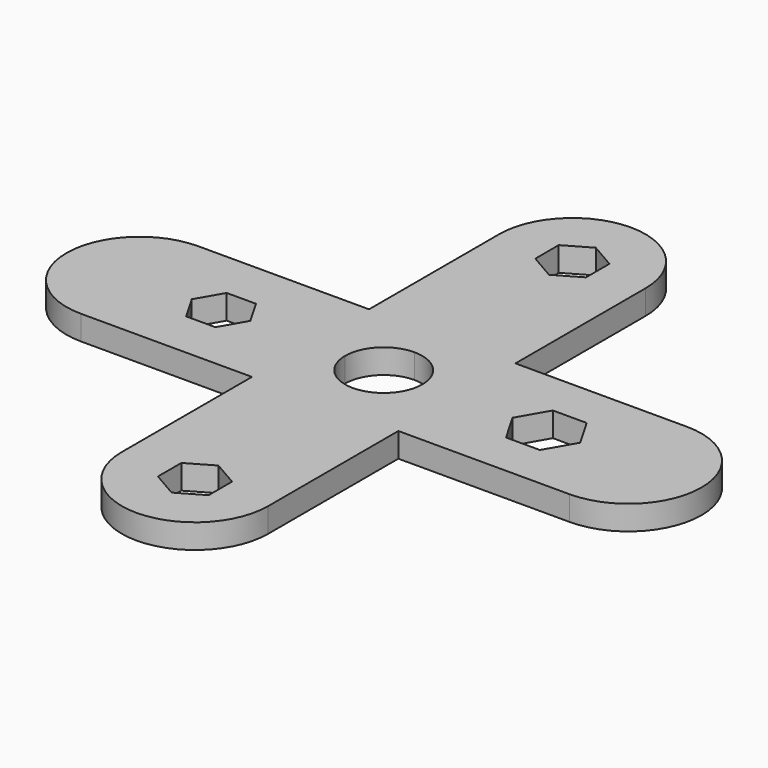
from build123d import *

# Parameters (mm, degrees)
F1_DEPTH = 6


with BuildPart() as f1:
    # F0 (on Top) → F1 (new body)
    with BuildSketch(Plane.XY):
        with BuildLine():
            Line((18, 0), (9.5, 0))
            ThreePointArc((9.5, 0), (6.7175144213, -6.7175144213), (0, -9.5))
            Line((0, -9.5), (0, -18))
            Line((0, -18), (18, -18))
            Line((18, -18), (40, -18))
            Line((40, -18), (60.1537041366, -18))
            ThreePointArc((60.1537041366, -18), (78.1537041366, 0), (60.1537041366, 18))
            Line((60.1537041366, 18), (40, 18))
            Line((40, 18), (18, 18))
            Line((18, 18), (18, 0))
        make_face()
        Polygon((35.8430780618, -7.2), (31.6861561237, 0), (35.8430780618, 7.2), (44.1569219382, 7.2), (48.3138438763, 0), (44.1569219382, -7.2), align=None, mode=Mode.SUBTRACT)
        with BuildLine():
            ThreePointArc((0, 9.5), (6.7175144213, 6.7175144213), (9.5, 0))
            Line((9.5, 0), (18, 0))
            Line((18, 0), (18, 18))
            Line((18, 18), (0, 18))
            Line((0, 18), (0, 9.5))
        make_face()
        with BuildLine():
            ThreePointArc((-9.5, 0), (-6.7175144213, 6.7175144213), (0, 9.5))
            Line((0, 9.5), (0, 18))
            Line((0, 18), (-18, 18))
            Line((-18, 18), (-18, 0))
            Line((-18, 0), (-9.5, 0))
        make_face()
        with BuildLine():
            Line((0, -18), (0, -9.5))
            ThreePointArc((0, -9.5), (-6.7175144213, -6.7175144213), (-9.5, 0))
            Line((-9.5, 0), (-18, 0))
            Line((-18, 0), (-18, -18))
            Line((-18, -18), (0, -18))
        make_face()
        Polygon((0, 40), (0, 18), (18, 18), (18, 58), (6.2353829072, 58), (6.2353829072, 54.4), (0, 50.8), align=None)
        Polygon((-18, 18), (0, 18), (0, 40), (0, 50.8), (-6.2353829072, 54.4), (-6.2353829072, 58), (-18, 58), (-18, 40), align=None)
        Polygon((0, -50.8), (0, -18), (-18, -18), (-18, -58), (-6.2353829072, -58), (-6.2353829072, -54.4), align=None)
        Polygon((18, -18), (0, -18), (0, -50.8), (6.2353829072, -54.4), (6.2353829072, -58), (18, -58), align=None)
        with BuildLine():
            Line((-18, -18), (-18, 0))
            Line((-18, 0), (-18, 18))
            Line((-18, 18), (-40, 18))
            Line((-40, 18), (-60, 18))
            ThreePointArc((-60, 18), (-78, 0), (-60, -18))
            Line((-60, -18), (-40, -18))
            Line((-40, -18), (-18, -18))
        make_face()
        Polygon((-36.4, 6.2353829072), (-32.8, 0), (-36.4, -6.2353829072), (-43.6, -6.2353829072), (-47.2, 0), (-43.6, 6.2353829072), align=None, mode=Mode.SUBTRACT)
        with BuildLine():
            Line((6.2353829072, 58), (18, 58))
            ThreePointArc((18, 58), (0, 76), (-18, 58))
            Line((-18, 58), (-6.2353829072, 58))
            Line((-6.2353829072, 58), (-6.2353829072, 61.6))
            Line((-6.2353829072, 61.6), (0, 65.2))
            Line((0, 65.2), (6.2353829072, 61.6))
            Line((6.2353829072, 61.6), (6.2353829072, 58))
        make_face()
        with BuildLine():
            Line((-6.2353829072, -58), (-18, -58))
            ThreePointArc((-18, -58), (0, -76), (18, -58))
            Line((18, -58), (6.2353829072, -58))
            Line((6.2353829072, -58), (6.2353829072, -61.6))
            Line((6.2353829072, -61.6), (0, -65.2))
            Line((0, -65.2), (-6.2353829072, -61.6))
            Line((-6.2353829072, -61.6), (-6.2353829072, -58))
        make_face()
    extrude(amount=F1_DEPTH)


solid = f1.part
